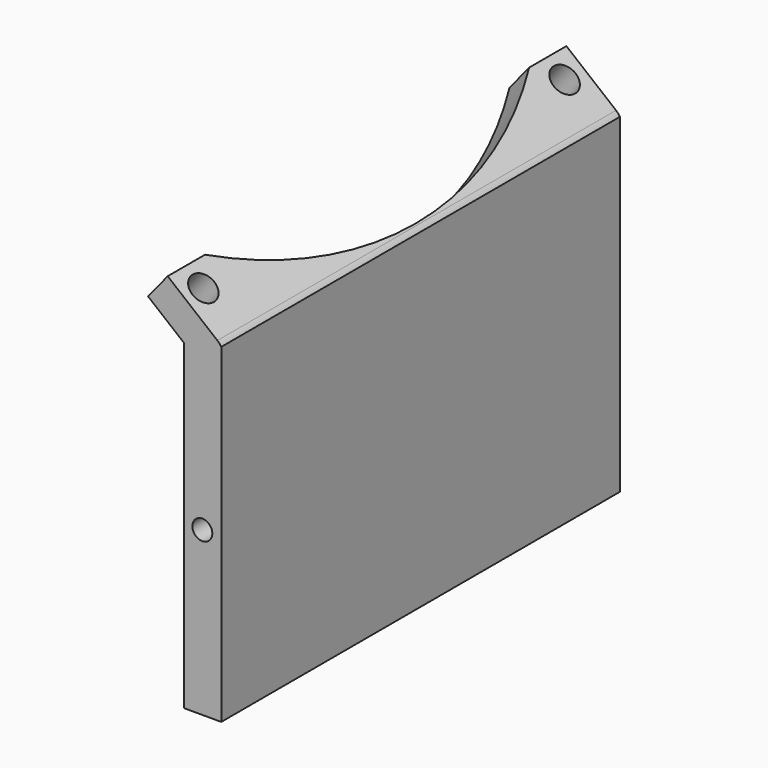
from build123d import *

# Parameters (mm, degrees)
F1_DEPTH      = 40
F2_DEPTH      = 50
F3_R          = 2.2048801609
F3_R_2        = 2.1982432021
F4_DEPTH      = 28.8
F4_DEPTH_BACK = 25
F5_W          = 10.2
F5_H          = 80
F6_DEPTH      = 24.9
F7_T1_DEPTH   = 85.5665416349
F8_W          = 80
F8_H          = 50
F9_DEPTH      = 2
F11_DEPTH     = 80
F13_DEPTH     = 25
F14_R         = 1.6
F15_DEPTH     = 5
F16_R         = 1.6
F17_DEPTH     = 5


# Not quite as in the source:
# - a fillet or chamfer that OpenCascade refuses, or shapes differently, is made with other operations: its cross-section is extruded or revolved along the edge and cut away or added
# - a feature names something its author has since deleted; it is built from what else it names


with BuildPart() as f1:
    # F0 (on Front) → F1 (new body, symmetric)
    with BuildSketch(Plane.XZ):
        Polygon((-7.7554572706, 6.3129139487), (0, 0), (4, 0), (4, 3), (4.2347525098, 3), (-4.5990002963, 10.190642584), align=None)
    extrude(amount=F1_DEPTH, both=True)

    # F2 (add): a face of the model
    f2_faces = [f1.faces().sort_by_distance(p)[0] for p in [
        (2, 0, 0),
    ]]
    extrude(f2_faces, amount=F2_DEPTH)

    # F3 (on face) → F4 (cut, two sides)
    with BuildSketch(Plane(origin=(0, 0, 0), x_dir=(0.7755457271, 0, -0.6312913949), z_dir=(-0.6312913949, 0, -0.7755457271))) as f4_sk:
        with BuildLine():
            ThreePointArc((-10, -32.5242628716), (-2.5564454764, -17.0134334817), (0, 0))
            ThreePointArc((0, 0), (-2.5564454764, 17.0134334817), (-10, 32.5242628716))
            Line((-10, 32.5242628716), (-10, -32.5242628716))
        make_face()
        with Locations((-6.3940989785, -36.1467376351)):
            Circle(F3_R)
        with Locations((-6.3940975815, 36.3416559994)):
            Circle(F3_R_2)
    extrude(amount=-F4_DEPTH, mode=Mode.SUBTRACT)
    extrude(f4_sk.sketch, amount=F4_DEPTH_BACK, mode=Mode.SUBTRACT)

    # F5 (on face) → F6 (cut)
    with BuildSketch(Plane(origin=(0, 0, -50), x_dir=(1, 0, 0), z_dir=(0, 0, -1))):
        with Locations((9.4639954135, 0)):
            Rectangle(F5_W, F5_H)
    extrude(amount=-F6_DEPTH, mode=Mode.SUBTRACT)

    # F7: fillet of radius 3 on 1 edges, made by hand

    # F7_s2 → F7_t1 (cut)
    with BuildSketch(Plane.XZ.offset(-42.7832708174)):
        with BuildLine():
            ThreePointArc((3.3713309939, 3.7028219666), (3.7134521777, 3.3762659619), (4, 3))
            Line((4, 3), (4.2347525098, 3))
            Line((4.2347525098, 3), (3.3713309939, 3.7028219666))
        make_face()
    extrude(amount=F7_T1_DEPTH, mode=Mode.SUBTRACT)

    # F8 (on face) → F9 (join)
    with BuildSketch(Plane(origin=(0, 0, 0), x_dir=(0, -1, 0), z_dir=(-1, 0, 0))):
        with Locations((0, -25)):
            Rectangle(F8_W, F8_H)
        Polygon((0, 0), (-40, 0), (-40, -50), (40, -50), (40, 0), align=None)
    extrude(amount=F9_DEPTH)

    # F10 (on face) → F11 (join)
    with BuildSketch(Plane.XZ.offset(40)):
        Polygon((-2, 1.6279927097), (-2, 0), (0, 0), align=None)
    extrude(amount=-F11_DEPTH)

    # F12: union 

    # F13 (cut): a face of the model
    f13_faces = [f1.faces().sort_by_distance(p)[0] for p in [
        (-1.1984527779, 0, 0.9755361927),
    ]]
    extrude(f13_faces, amount=-F13_DEPTH, mode=Mode.SUBTRACT)

    # F14 (on face) → F15 (cut)
    with BuildSketch(Plane(origin=(0, 40, 0), x_dir=(-1, 0, 0), z_dir=(0, 1, 0))):
        with Locations((-0.9606604144, -23.8474996724)):
            Circle(F14_R)
    extrude(amount=-F15_DEPTH, mode=Mode.SUBTRACT)

    # F16 (on face) → F17 (cut)
    with BuildSketch(Plane.XZ.offset(40)):
        with Locations((0.9606604144, -23.8474996724)):
            Circle(F16_R)
    extrude(amount=-F17_DEPTH, mode=Mode.SUBTRACT)


solid = f1.part
